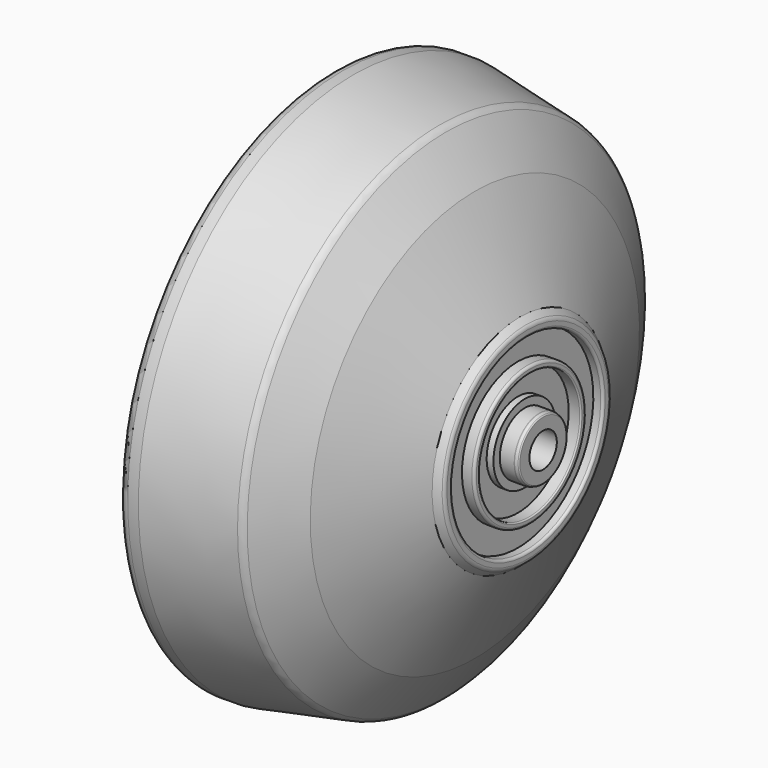
from build123d import *

# Parameters (mm, degrees)
F2_R = 1
F3_R = 0.5
F4_R = 1
F5_R = 1
F6_R = 2
F7_R = 2


# Not quite as in the source:
# - ends of sketch curves that miss each other by under 0.0002 mm in the source are joined


with BuildPart() as f1:
    # F0 (on Front) → F1 (revolve)
    with BuildSketch(Plane.XZ):
        with BuildLine():
            Line((1.054421, 1.754851), (4.24833, 1.754851))
            Line((4.24833, 1.754851), (4.24833, 2.965108))
            ThreePointArc((4.24833, 2.965108), (4.2243561549, 3.0393632641), (4.1614868664, 3.085580599))
            Line((4.1614868664, 3.085580599), (3.879268, 3.179662))
            ThreePointArc((3.879268, 3.179662), (3.8594525644, 3.1845473579), (3.83911, 3.18619))
            Line((3.83911, 3.18619), (2.36708, 3.18619))
            Line((2.36708, 3.18619), (2.36708, 3.998))
            Line((2.36708, 3.998), (1.672421, 3.998))
            Line((1.672421, 3.998), (1.672421, 6.492))
            Line((1.672421, 6.492), (2.801421, 6.492))
            ThreePointArc((2.801421, 6.492), (2.8912235612, 6.5291974388), (2.928421, 6.619))
            Line((2.928421, 6.619), (2.928421, 6.896))
            ThreePointArc((2.928421, 6.896), (2.8540261224, 7.0756051224), (2.674421, 7.15))
            Line((2.674421, 7.15), (1.668421, 7.15))
            Line((1.668421, 7.15), (1.668421, 7.150491))
            Line((1.668421, 7.150491), (1.668421, 9.65))
            Line((1.668421, 9.65), (1.668421, 9.65036))
            Line((1.668421, 9.65036), (2.419171, 9.651342))
            ThreePointArc((2.419171, 9.651342), (2.5987761224, 9.7257368776), (2.673171, 9.905342))
            Line((2.673171, 9.905342), (2.673171, 10.5649959296))
            Line((2.673171, 10.5649959296), (1.8690302968, 11.2215802073))
            Line((1.8690302968, 11.2215802073), (-2.7342122048, 21.0461560637))
            Line((-2.7342122048, 21.0461560637), (-5.9062168002, 25.7854051888))
            Line((-5.9062168002, 25.7854051888), (-15.1567570865, 27.5))
            Line((-15.1567570865, 27.5), (-17.25167, 27.5))
            Line((-17.25167, 27.5), (-17.25167, 26.0251207387))
            Line((-17.25167, 26.0251207387), (-17.25167, 25.0174365938))
            Line((-17.25167, 25.0174365938), (-12.6095786691, 24.157021368))
            Line((-12.6095786691, 24.157021368), (-11.5705328062, 23.9002071321))
            Line((-11.5705328062, 23.9002071321), (-11.5705328062, 20.409735066))
            Line((-11.5705328062, 20.409735066), (-10.5314869434, 20.409735066))
            Line((-10.5314869434, 20.409735066), (-4.0925083116, 20.409735066))
            Line((-4.0925083116, 20.409735066), (0, 11.6752053653))
            Line((0, 11.6752053653), (0, 8.8895335793))
            ThreePointArc((0, 8.8895335793), (-0.573002805, 7.2498007699), (-2.0425822586, 6.3238460571))
            ThreePointArc((-2.0425822586, 6.3238460571), (-1.7130561539, 3.1700482919), (-1.636756584, 0))
            Line((-1.636756584, 0), (0, 0))
            Line((0, 0), (1.054421, 1.754851))
        make_face()
    revolve(axis=Axis((-0.818378292, 0, 0), (-1, 0, 0)))

    # F2
    f2_edges = [f1.edges().sort_by_distance(p)[0] for p in [
        (-17.25167, 0, -27.5),
        (-17.25167, 0, -25.017437),
    ]]
    fillet(f2_edges, radius=F2_R)

    # F3
    f3_edges = [f1.edges().sort_by_distance(p)[0] for p in [
        (2.673171, 0, -10.564996),
    ]]
    fillet(f3_edges, radius=F3_R)

    # F4
    f4_edges = [f1.edges().sort_by_distance(p)[0] for p in [
        (-5.906217, 0, -25.785405),
    ]]
    fillet(f4_edges, radius=F4_R)

    # F5
    f5_edges = [f1.edges().sort_by_distance(p)[0] for p in [
        (-11.570533, 0, -20.409735),
    ]]
    fillet(f5_edges, radius=F5_R)

    # F6
    f6_edges = [f1.edges().sort_by_distance(p)[0] for p in [
        (-4.092508, 0, -20.409735),
        (0, 0, -11.675205),
    ]]
    fillet(f6_edges, radius=F6_R)

    # F7
    f7_edges = [f1.edges().sort_by_distance(p)[0] for p in [
        (-2.042582, 0, -6.323846),
    ]]
    fillet(f7_edges, radius=F7_R)


solid = f1.part
